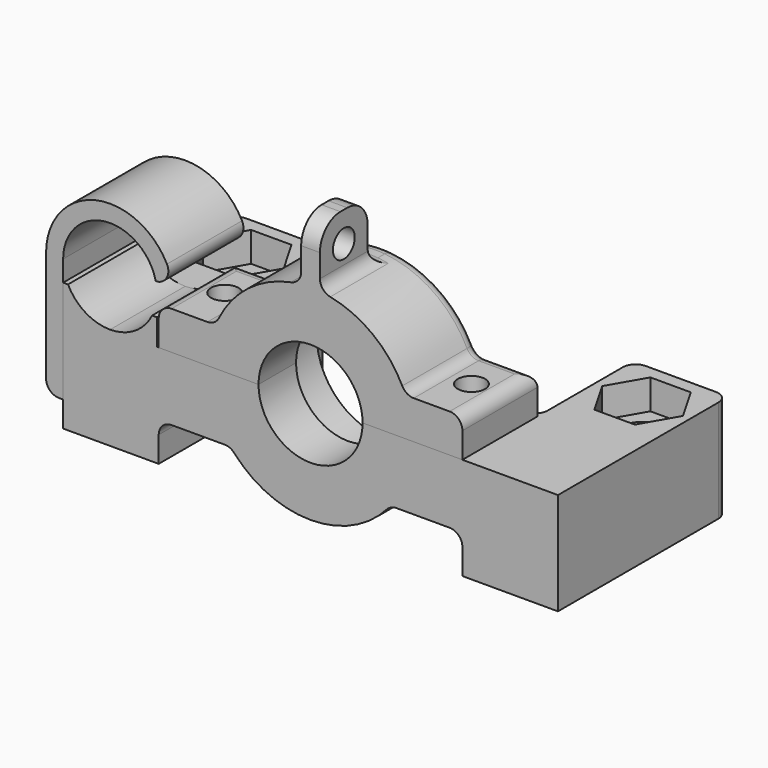
from build123d import *

# Parameters (mm, degrees)
F0_R          = 2.6
F1_DEPTH      = 12
F3_DEPTH      = 25
F4_DEPTH      = 11
F5_DEPTH      = 5.5
F6_DEPTH      = 11
F7_DEPTH      = 11
F8_R          = 1.4
F9_DEPTH      = 25
F8_R_2        = 1.6
F10_DEPTH     = 5
F11_R         = 1.0512240851
F12_DEPTH     = 8
F13_DEPTH     = 2.2
F15_DEPTH     = 4
F16_R         = 1.6
F17_DEPTH     = 3
F18_T1_DEPTH  = 11
F18_T3_DEPTH  = 7
F18_T8_ANGLE  = 46.3290515764
F18_T15_DEPTH = 10.2444672311
F18_T19_ANGLE = 46.3290515764
F18_T26_DEPTH = 10.2444672311
F18_T30_ANGLE = 46.3290515764
F18_F33_R     = 1.5
F19_R         = 3
F20_R         = 2.6
F21_DEPTH     = 3.5
F22_R         = 1.5
F24_DEPTH     = 5
F25_T1_DEPTH  = 22.5249918974
F25_T3_DEPTH  = 18.5
F26_R         = 1.5


# Not quite as in the source:
# - a fillet or chamfer that OpenCascade refuses, or shapes differently, is made with other operations: its cross-section is extruded or revolved along the edge and cut away or added


with BuildPart() as f1:
    # F0 (on Top) → F1 (new body)
    with BuildSketch(Plane.XY):
        Polygon((17.8, 0), (0, 0), (-17.8, 0), (-17.8, 14), (-29, 14), (-29, -11), (0, -11), (29, -11), (29, 14), (17.8, 14), align=None)
        with Locations((-23.4, 8.4)):
            Circle(F0_R, mode=Mode.SUBTRACT)
        with Locations((23.4, 8.4)):
            Circle(F0_R, mode=Mode.SUBTRACT)
    extrude(amount=F1_DEPTH)

    # F2 (on face) → F3 (cut)
    with BuildSketch(Plane(origin=(0, 0, 0), x_dir=(-1, 0, 0), z_dir=(0, 1, 0))):
        with BuildLine():
            Line((17.8, 4.5), (9.3674969976, 4.5))
            ThreePointArc((9.3674969976, 4.5), (5.1961524227, 1.1833461736), (0, 0))
            Line((0, 0), (17.8, 0))
            Line((17.8, 0), (17.8, 4.5))
        make_face()
        with BuildLine():
            ThreePointArc((0, 0), (-5.1961524227, 1.1833461736), (-9.3674969976, 4.5))
            Line((-9.3674969976, 4.5), (-17.8, 4.5))
            Line((-17.8, 4.5), (-17.8, 0))
            Line((-17.8, 0), (0, 0))
        make_face()
        with BuildLine():
            ThreePointArc((-6.1, 12), (0, 5.9), (6.1, 12))
            Line((6.1, 12), (-6.1, 12))
        make_face()
    extrude(amount=-F3_DEPTH, mode=Mode.SUBTRACT)


with BuildPart() as f4:
    # F2 (on face) → F4 (new body)
    with BuildSketch(Plane(origin=(0, 0, 0), x_dir=(-1, 0, 0), z_dir=(0, 1, 0))):
        with BuildLine():
            ThreePointArc((11.1242977306, 16.5), (11.77904013, 14.2922071495), (12, 12))
            Line((12, 12), (12.6856295392, 12))
            Line((12.6856295392, 12), (17.8, 12))
            Line((17.8, 12), (17.8, 16.5))
            Line((17.8, 16.5), (11.1242977306, 16.5))
        make_face()
        with BuildLine():
            ThreePointArc((-8.1, 12), (0, 20.1), (8.1, 12))
            Line((8.1, 12), (12, 12))
            ThreePointArc((12, 12), (11.77904013, 14.2922071495), (11.1242977306, 16.5))
            ThreePointArc((11.1242977306, 16.5), (7.1576560797, 21.6316125049), (1.1, 23.949476976))
            ThreePointArc((1.1, 23.949476976), (0, 24), (-1.1, 23.949476976))
            ThreePointArc((-1.1, 23.949476976), (-7.1576560797, 21.6316125049), (-11.1242977306, 16.5))
            ThreePointArc((-11.1242977306, 16.5), (-11.77904013, 14.2922071495), (-12, 12))
            Line((-12, 12), (-8.1, 12))
        make_face()
        with BuildLine():
            ThreePointArc((-6.1, 12), (0, 18.1), (6.1, 12))
            Line((6.1, 12), (8.1, 12))
            ThreePointArc((8.1, 12), (0, 20.1), (-8.1, 12))
            Line((-8.1, 12), (-6.1, 12))
        make_face()
        with BuildLine():
            Line((-17.8, 12), (-12, 12))
            ThreePointArc((-12, 12), (-11.77904013, 14.2922071495), (-11.1242977306, 16.5))
            Line((-11.1242977306, 16.5), (-17.8, 16.5))
            Line((-17.8, 16.5), (-17.8, 12))
        make_face()
        with BuildLine():
            ThreePointArc((-1.1, 23.949476976), (0, 24), (1.1, 23.949476976))
            Line((1.1, 23.949476976), (1.1, 30.949476976))
            Line((1.1, 30.949476976), (0, 30.949476976))
            Line((0, 30.949476976), (-1.1, 30.949476976))
            Line((-1.1, 30.949476976), (-1.1, 23.949476976))
        make_face()
    extrude(amount=-F4_DEPTH)


with BuildPart() as f5_tool:
    # F2 (on face) → F5 (new body)
    with BuildSketch(Plane(origin=(0, 0, 0), x_dir=(-1, 0, 0), z_dir=(0, 1, 0))):
        with BuildLine():
            Line((8.1, 12), (6.1, 12))
            ThreePointArc((6.1, 12), (0, 5.9), (-6.1, 12))
            Line((-6.1, 12), (-8.1, 12))
            ThreePointArc((-8.1, 12), (0, 3.9), (8.1, 12))
        make_face()
        with BuildLine():
            ThreePointArc((-6.1, 12), (0, 18.1), (6.1, 12))
            Line((6.1, 12), (8.1, 12))
            ThreePointArc((8.1, 12), (0, 20.1), (-8.1, 12))
            Line((-8.1, 12), (-6.1, 12))
        make_face()
    extrude(amount=-F5_DEPTH)


with BuildPart() as f1_1:
    add(f1.part)

    # F5: cut by f5_tool
    add(f5_tool.part, mode=Mode.SUBTRACT)

    # F2 (on face) → F7 (join)
    with BuildSketch(Plane(origin=(0, 0, 0), x_dir=(-1, 0, 0), z_dir=(0, 1, 0))):
        with BuildLine():
            ThreePointArc((28.4295173729, 15.0607668274), (26.4012254056, 12.8274320609), (23.500000032, 12))
            Line((23.500000032, 12), (29, 12))
            Line((29, 12), (29, 15.0607668274))
            Line((29, 15.0607668274), (28.4295173729, 15.0607668274))
        make_face()
        with BuildLine():
            Line((18, 15.0607668274), (18, 12))
            Line((18, 12), (23.500000032, 12))
            ThreePointArc((23.500000032, 12), (20.5987746216, 12.827432044), (18.5704826271, 15.0607668274))
            Line((18.5704826271, 15.0607668274), (18, 15.0607668274))
        make_face()
    extrude(amount=-F7_DEPTH)


with BuildPart() as f4_1:
    add(f4.part)

    # F5: cut by f5_tool
    add(f5_tool.part, mode=Mode.SUBTRACT)


with BuildPart() as f6:
    # F2 (on face) → F6 (new body)
    with BuildSketch(Plane(origin=(0, 0, 0), x_dir=(-1, 0, 0), z_dir=(0, 1, 0))):
        with BuildLine():
            Line((29, 4.521176219), (29, 3))
            Line((29, 3), (31, 3))
            Line((31, 3), (31, 17.5))
            ThreePointArc((31, 17.5), (24.1260825887, 24.9738223549), (16.1045278421, 18.7477946793))
            Line((16.1045278421, 18.7477946793), (18.1434144795, 18.7477946793))
            ThreePointArc((18.1434144795, 18.7477946793), (24.1280046327, 22.96402875), (29, 17.5))
            Line((29, 17.5), (29, 17.4876172096))
            Line((29, 17.4876172096), (29, 15.0607668274))
            Line((29, 15.0607668274), (29, 12))
            Line((29, 12), (29, 4.521176219))
        make_face()
    extrude(amount=-F6_DEPTH)


with BuildPart() as f9_tool:
    # F8 (on face) → F9 (new body)
    with BuildSketch(Plane.XY.offset(16.5)):
        with Locations((14.4621488653, -5.5)):
            Circle(F8_R)
        with Locations((-14.4621488653, -5.5)):
            Circle(F8_R)
    extrude(amount=-F9_DEPTH)


with BuildPart() as f1_2:
    add(f1_1.part)

    # F9: cut by f9_tool
    add(f9_tool.part, mode=Mode.SUBTRACT)


with BuildPart() as f4_2:
    add(f4_1.part)

    # F9: cut by f9_tool
    add(f9_tool.part, mode=Mode.SUBTRACT)

    # F8 (on face) → F10 (cut)
    with BuildSketch(Plane.XY.offset(16.5)):
        with Locations((-14.4621488653, -5.5)):
            Circle(F8_R_2)
        with Locations((-14.4621488653, -5.5)):
            Circle(F8_R, mode=Mode.SUBTRACT)
        with Locations((14.4621488653, -5.5)):
            Circle(F8_R_2)
        with Locations((14.4621488653, -5.5)):
            Circle(F8_R, mode=Mode.SUBTRACT)
    extrude(amount=-F10_DEPTH, mode=Mode.SUBTRACT)

    # F2 (on face) → F15 (cut)
    with BuildSketch(Plane(origin=(0, 0, 0), x_dir=(-1, 0, 0), z_dir=(0, 1, 0))):
        with BuildLine():
            ThreePointArc((-1.1, 23.949476976), (0, 24), (1.1, 23.949476976))
            Line((1.1, 23.949476976), (1.1, 30.949476976))
            Line((1.1, 30.949476976), (0, 30.949476976))
            Line((0, 30.949476976), (-1.1, 30.949476976))
            Line((-1.1, 30.949476976), (-1.1, 23.949476976))
        make_face()
    extrude(amount=-F15_DEPTH, mode=Mode.SUBTRACT)

    # F16 (on face) → F17 (cut)
    with BuildSketch(Plane.YZ.offset(1.1)):
        with Locations((-7.5, 27.449476976)):
            Circle(F16_R)
    extrude(amount=-F17_DEPTH, mode=Mode.SUBTRACT)

    # F18: fillet of radius 1.5 on 8 edges, made by hand

    # F18_s2 → F18_t1 (join)
    with BuildSketch(Plane.XZ):
        with BuildLine():
            ThreePointArc((-12.0933866224, 16.5), (-11.3028172074, 16.7252451216), (-10.7496769977, 17.3333333333))
            Line((-10.7496769977, 17.3333333333), (-10.7228028052, 17.32))
            ThreePointArc((-10.7228028052, 17.32), (-10.9175590629, 16.9079327733), (-11.0964869863, 16.48875))
            Line((-11.0964869863, 16.48875), (-11.1242977306, 16.47))
            Line((-11.1242977306, 16.47), (-12.0933866224, 16.47))
            Line((-12.0933866224, 16.47), (-12.0933866224, 16.5))
        make_face()
        with BuildLine():
            ThreePointArc((12.0933866224, 16.5), (11.3028172074, 16.7252451216), (10.7496769977, 17.3333333333))
            Line((10.7496769977, 17.3333333333), (10.7228028052, 17.32))
            ThreePointArc((10.7228028052, 17.32), (10.9175590629, 16.9079327733), (11.0964869863, 16.48875))
            Line((11.0964869863, 16.48875), (11.1242977306, 16.47))
            Line((11.1242977306, 16.47), (12.0933866224, 16.47))
            Line((12.0933866224, 16.47), (12.0933866224, 16.5))
        make_face()
    extrude(amount=F18_T1_DEPTH)

    # F18_s4 → F18_t3 (join)
    with BuildSketch(Plane.XZ.offset(4)):
        with BuildLine():
            ThreePointArc((2.3111111111, 23.7753456608), (1.4416966431, 24.2941986381), (1.1, 25.2472638684))
            Line((1.1, 25.2472638684), (1.07, 25.2472638684))
            Line((1.07, 25.2472638684), (1.07, 23.949476976))
            Line((1.07, 23.949476976), (1.09725, 23.9196032836))
            ThreePointArc((1.09725, 23.9196032836), (1.7035069442, 23.8481628994), (2.3053333333, 23.7459072967))
            Line((2.3053333333, 23.7459072967), (2.3111111111, 23.7753456608))
        make_face()
        with BuildLine():
            ThreePointArc((-2.3111111111, 23.7753456608), (-1.4416966431, 24.2941986381), (-1.1, 25.2472638684))
            Line((-1.1, 25.2472638684), (-1.07, 25.2472638684))
            Line((-1.07, 25.2472638684), (-1.07, 23.949476976))
            Line((-1.07, 23.949476976), (-1.09725, 23.9196032836))
            ThreePointArc((-1.09725, 23.9196032836), (-1.7035069442, 23.8481628994), (-2.3053333333, 23.7459072967))
            Line((-2.3053333333, 23.7459072967), (-2.3111111111, 23.7753456608))
        make_face()
    extrude(amount=F18_T3_DEPTH)


with BuildPart() as f12_tool:
    # F11 (on face) → F12 (new body)
    with BuildSketch(Plane(origin=(-31, 0, 0), x_dir=(0, -1, 0), z_dir=(-1, 0, 0))):
        with Locations((8.030994951, 9.7125562447)):
            Circle(F11_R)
        with Locations((2.969005049, 9.7125562447)):
            Circle(F11_R)
    extrude(amount=-F12_DEPTH)


with BuildPart() as f1_3:
    add(f1_2.part)

    # F12: cut by f12_tool
    add(f12_tool.part, mode=Mode.SUBTRACT)

    # F20 (on face) → F21 (cut)
    with BuildSketch(Plane.XY.offset(12)):
        Polygon((21.0328638963, 4.3), (25.7671361037, 4.3), (28.1342722074, 8.4), (25.7671361037, 12.5), (21.0328638963, 12.5), (18.6657277926, 8.4), align=None)
        with Locations((23.4, 8.4)):
            Circle(F20_R, mode=Mode.SUBTRACT)
        Polygon((-18.6657277926, 8.4), (-21.0328638963, 12.5), (-25.7671361037, 12.5), (-28.1342722074, 8.4), (-25.7671361037, 4.3), (-21.0328638963, 4.3), align=None)
    extrude(amount=-F21_DEPTH, mode=Mode.SUBTRACT)

    # F22
    f22_edges = [f1_3.edges().sort_by_distance(p)[0] for p in [
        (-29, 14, 6),
        (-17.8, 14, 6),
        (17.8, 14, 6),
        (29, 14, 6),
    ]]
    fillet(f22_edges, radius=F22_R)

    # F23 (on face) → F24 (cut)
    with BuildSketch(Plane(origin=(0, 14, 0), x_dir=(-1, 0, 0), z_dir=(0, 1, 0))):
        with BuildLine():
            Line((27.5, 2.9973696215), (27.5, 3.2668135832))
            ThreePointArc((27.5, 3.2668135832), (25.3082811773, 3.1320916023), (27.5, 2.9973696215))
        make_face()
    extrude(amount=-F24_DEPTH, mode=Mode.SUBTRACT)

    # F26
    f26_edges = [f1_3.edges().sort_by_distance(p)[0] for p in [
        (-17.8, 0, 8.25),
        (17.8, 0, 8.25),
        (-17.8, -5.5, 4.5),
        (-9.367497, -5.5, 4.5),
        (9.367497, -5.5, 4.5),
        (17.8, -5.5, 4.5),
        (-13.583748, 0, 4.5),
        (0, 0, 0),
        (13.583748, 0, 4.5),
    ]]
    fillet(f26_edges, radius=F26_R)


with BuildPart() as f6_1:
    add(f6.part)

    # F12: cut by f12_tool
    add(f12_tool.part, mode=Mode.SUBTRACT)

    # F11 (on face) → F13 (cut)
    with BuildSketch(Plane(origin=(-31, 0, 0), x_dir=(0, -1, 0), z_dir=(-1, 0, 0))):
        with BuildLine():
            Line((9.290994951, 9.7125562447), (9.290994951, 12.2325562447))
            ThreePointArc((9.290994951, 12.2325562447), (8.030994951, 13.4925562447), (6.770994951, 12.2325562447))
            Line((6.770994951, 12.2325562447), (6.770994951, 9.7125562447))
            Line((6.770994951, 9.7125562447), (6.7729224477, 7.3787025467))
            Line((6.7729224477, 7.3787025467), (6.7730392388, 7.2372893661))
            ThreePointArc((6.7730392388, 7.2372893661), (8.0322897625, 6.0490355977), (9.2890954617, 7.2398749377))
            Line((9.2890954617, 7.2398749377), (9.2892002329, 7.376261926))
            Line((9.2892002329, 7.376261926), (9.290994951, 9.7125562447))
        make_face()
        with Locations((8.030994951, 9.7125562447)):
            Circle(F11_R, mode=Mode.SUBTRACT)
        with BuildLine():
            ThreePointArc((4.229005049, 12.2325562447), (2.969005049, 13.4925562447), (1.709005049, 12.2325562447))
            Line((1.709005049, 12.2325562447), (1.709005049, 9.7125562447))
            Line((1.709005049, 9.7125562447), (1.7107997671, 7.376261926))
            Line((1.7107997671, 7.376261926), (1.7109045383, 7.2398749377))
            ThreePointArc((1.7109045383, 7.2398749377), (2.9677102375, 6.0490355977), (4.2269607612, 7.2372893661))
            Line((4.2269607612, 7.2372893661), (4.2270775523, 7.3787025467))
            Line((4.2270775523, 7.3787025467), (4.229005049, 9.7125562447))
            Line((4.229005049, 9.7125562447), (4.229005049, 12.2325562447))
        make_face()
        with Locations((2.969005049, 9.7125562447)):
            Circle(F11_R, mode=Mode.SUBTRACT)
    extrude(amount=-F13_DEPTH, mode=Mode.SUBTRACT)

    # F25: fillet of radius 1.5 on 2 edges, made by hand

    # F25_s2 → F25_t1 (cut)
    with BuildSketch(Plane.XZ.offset(-5.7624959487)):
        with BuildLine():
            ThreePointArc((-18.1661810679, 18.7477946793), (-16.8854736453, 19.466905124), (-16.8327263349, 20.9347433492))
            ThreePointArc((-16.8327263349, 20.9347433492), (-16.3841099544, 19.8694110784), (-16.1045278421, 18.7477946793))
            Line((-16.1045278421, 18.7477946793), (-18.1661810679, 18.7477946793))
        make_face()
    extrude(amount=F25_T1_DEPTH, mode=Mode.SUBTRACT)

    # F25_s4 → F25_t3 (cut)
    with BuildSketch(Plane.XZ.offset(-3.75)):
        with BuildLine():
            ThreePointArc((-29.5, 3), (-30.5606601718, 3.4393398282), (-31, 4.5))
            Line((-31, 4.5), (-31, 3))
            Line((-31, 3), (-29.5, 3))
        make_face()
    extrude(amount=F25_T3_DEPTH, mode=Mode.SUBTRACT)


with BuildPart() as f18_tool6:
    # F18_s7 → F18_t8 (revolve)
    with BuildSketch(Plane(origin=(-4.3399041713, 0, 1.8569055304), x_dir=(0, 1, 0), z_dir=(0.919379069, 0, -0.393372759))):
        with BuildLine():
            ThreePointArc((-2.5, 23.0325488277), (-3.5606601718, 23.4718886559), (-4, 24.5325488277))
            Line((-4, 24.5325488277), (-4.03, 24.5325488277))
            Line((-4.03, 24.5325488277), (-4.03, 23.0025488277))
            Line((-4.03, 23.0025488277), (-2.5, 23.0025488277))
            Line((-2.5, 23.0025488277), (-2.5, 23.0325488277))
        make_face()
    revolve(axis=Axis((0, -4, 12), (0, -1, 0)), revolution_arc=F18_T8_ANGLE)

    split(bisect_by=Plane.YZ.offset(-1.1), keep=Keep.TOP)

    split(bisect_by=Plane.YZ.offset(1.1), keep=Keep.BOTTOM)


with BuildPart() as f4_3:
    add(f4_2.part)

    # F18_t5: union F18_tool6
    add(f18_tool6.part)


with BuildPart() as f18_tool13:
    # F18_s14 → F18_t15 (new body)
    with BuildSketch(Plane.XZ.offset(0.7555327689)):
        with BuildLine():
            ThreePointArc((2.3111111111, 23.7753456608), (1.4416966431, 24.2941986381), (1.1, 25.2472638684))
            Line((1.1, 25.2472638684), (1.07, 25.2472638684))
            Line((1.07, 25.2472638684), (1.07, 23.949476976))
            Line((1.07, 23.949476976), (1.09725, 23.9196032836))
            ThreePointArc((1.09725, 23.9196032836), (1.7035069442, 23.8481628994), (2.3053333333, 23.7459072967))
            Line((2.3053333333, 23.7459072967), (2.3111111111, 23.7753456608))
        make_face()
    extrude(amount=F18_T15_DEPTH)

    split(bisect_by=Plane.XZ.offset(4), keep=Keep.BOTTOM)


with BuildPart() as f18_tool17:
    # F18_s18 → F18_t19 (revolve)
    with BuildSketch(Plane(origin=(-4.3399041713, 0, 1.8569055304), x_dir=(0, 1, 0), z_dir=(0.919379069, 0, -0.393372759))):
        with BuildLine():
            ThreePointArc((-2.5, 23.0325488277), (-3.5606601718, 23.4718886559), (-4, 24.5325488277))
            Line((-4, 24.5325488277), (-4.03, 24.5325488277))
            Line((-4.03, 24.5325488277), (-4.03, 23.0025488277))
            Line((-4.03, 23.0025488277), (-2.5, 23.0025488277))
            Line((-2.5, 23.0025488277), (-2.5, 23.0325488277))
        make_face()
    revolve(axis=Axis((0, -4, 12), (0, -1, 0)), revolution_arc=F18_T19_ANGLE)

    split(bisect_by=Plane.YZ.offset(1.1), keep=Keep.TOP)


with BuildPart() as f18_tool13_1:
    add(f18_tool13.part)

    # F18_t21: intersect F18_tool17
    add(f18_tool17.part, mode=Mode.INTERSECT)


with BuildPart() as f4_4:
    add(f4_3.part)

    # F18_t11: union F18_tool13
    add(f18_tool13_1.part)


with BuildPart() as f18_tool24:
    # F18_s25 → F18_t26 (new body)
    with BuildSketch(Plane.XZ.offset(0.7555327689)):
        with BuildLine():
            ThreePointArc((-2.3111111111, 23.7753456608), (-1.4416966431, 24.2941986381), (-1.1, 25.2472638684))
            Line((-1.1, 25.2472638684), (-1.07, 25.2472638684))
            Line((-1.07, 25.2472638684), (-1.07, 23.949476976))
            Line((-1.07, 23.949476976), (-1.09725, 23.9196032836))
            ThreePointArc((-1.09725, 23.9196032836), (-1.7035069442, 23.8481628994), (-2.3053333333, 23.7459072967))
            Line((-2.3053333333, 23.7459072967), (-2.3111111111, 23.7753456608))
        make_face()
    extrude(amount=F18_T26_DEPTH)

    split(bisect_by=Plane.XZ.offset(4), keep=Keep.BOTTOM)


with BuildPart() as f18_tool28:
    # F18_s29 → F18_t30 (revolve)
    with BuildSketch(Plane(origin=(-4.3399041713, 0, 1.8569055304), x_dir=(0, 1, 0), z_dir=(0.919379069, 0, -0.393372759))):
        with BuildLine():
            ThreePointArc((-2.5, 23.0325488277), (-3.5606601718, 23.4718886559), (-4, 24.5325488277))
            Line((-4, 24.5325488277), (-4.03, 24.5325488277))
            Line((-4.03, 24.5325488277), (-4.03, 23.0025488277))
            Line((-4.03, 23.0025488277), (-2.5, 23.0025488277))
            Line((-2.5, 23.0025488277), (-2.5, 23.0325488277))
        make_face()
    revolve(axis=Axis((0, -4, 12), (0, -1, 0)), revolution_arc=F18_T30_ANGLE)

    split(bisect_by=Plane.YZ.offset(-1.1), keep=Keep.BOTTOM)


with BuildPart() as f18_tool24_1:
    add(f18_tool24.part)

    # F18_t32: intersect F18_tool28
    add(f18_tool28.part, mode=Mode.INTERSECT)


with BuildPart() as f4_5:
    add(f4_4.part)

    # F18_t22: union F18_tool24
    add(f18_tool24_1.part)

    # F18_f33
    f18_f33_edges = [f4_5.edges().sort_by_distance(p)[0] for p in [
        (-14.9466933112, 0, 16.5),
        (17.8, -5.5, 16.5),
        (-17.8, -5.5, 16.5),
        (-11.3028172074, 0, 16.7252451216),
    ]]
    fillet(f18_f33_edges, radius=F18_F33_R)

    # F19
    f19_edges = [f4_5.edges().sort_by_distance(p)[0] for p in [
        (0, -4, 30.949477),
        (0, -11, 30.949477),
    ]]
    fillet(f19_edges, radius=F19_R)


solid = Compound([f1_3.part, f6_1.part, f4_5.part])
